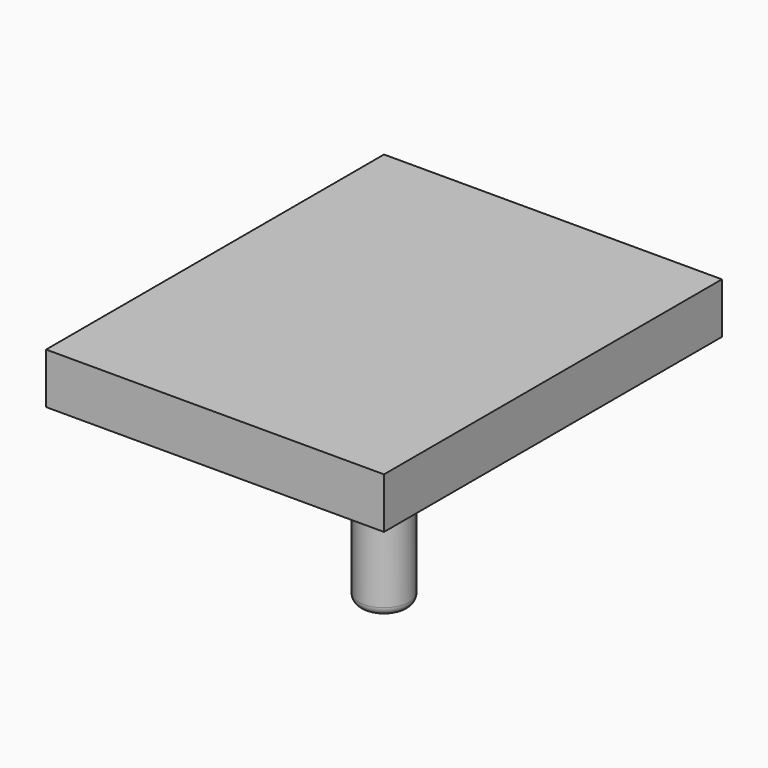
from build123d import *

# Parameters (mm, degrees)
F1_W     = 20
F1_H     = 25
F2_DEPTH = 3
F3_R     = 1.5
F4_DEPTH = 12
F0_R     = 0.5


with BuildPart() as f2:
    # F1 (on Top) → F2 (new body)
    with BuildSketch(Plane.XY):
        Rectangle(F1_W, F1_H)
    extrude(amount=F2_DEPTH)

    # F3 (on face) → F4 (join)
    with BuildSketch(Plane(origin=(0, 0, 0), x_dir=(1, 0, 0), z_dir=(0, 0, -1))):
        Circle(F3_R)
    extrude(amount=F4_DEPTH)

    # F0
    f0_edges = [f2.edges().sort_by_distance(p)[0] for p in [
        (-1.5, 0, -12),
    ]]
    fillet(f0_edges, radius=F0_R)


solid = f2.part
